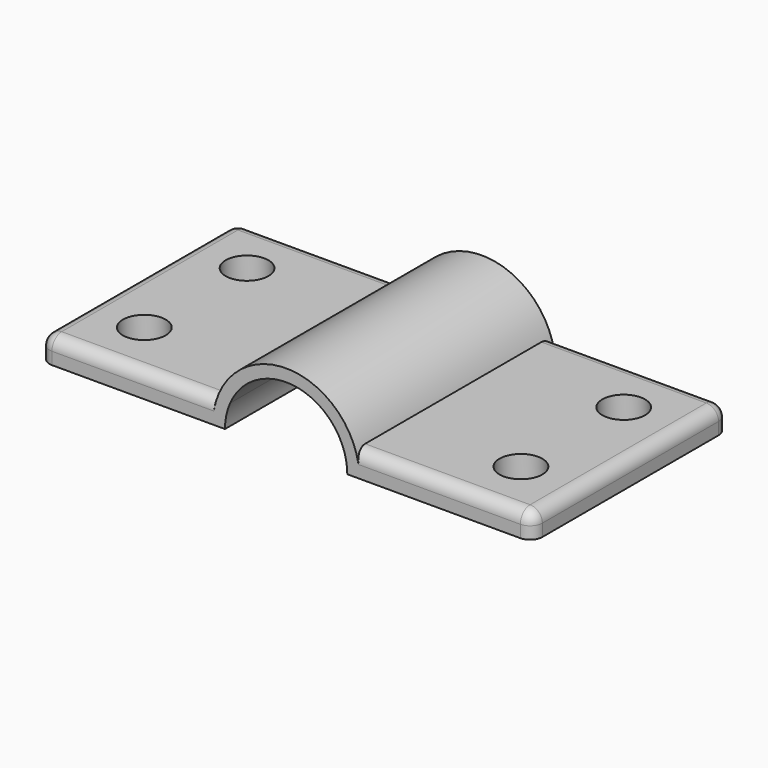
from build123d import *

# Parameters (mm, degrees)
F0_W         = 40.28548
F0_H         = 20
F0_R         = 1.75
F1_DEPTH     = 10
F3_DEPTH     = 25
F4_R         = 1
F5_T1_DEPTH  = 3.5
F5_S5_W      = 1
F5_S5_H      = 1
F5_T6_DEPTH  = 1
F5_S11_W     = 1
F5_S11_H     = 1
F5_T12_DEPTH = 1
F5_S17_W     = 1
F5_S17_H     = 1
F5_T18_DEPTH = 1
F5_S23_W     = 1
F5_S23_H     = 1
F5_T24_DEPTH = 1


# Not quite as in the source:
# - a fillet or chamfer that OpenCascade refuses, or shapes differently, is made with other operations: its cross-section is extruded or revolved along the edge and cut away or added


with BuildPart() as f1:
    # F0 (on Top) → F1 (new body)
    with BuildSketch(Plane.XY):
        Rectangle(F0_W, F0_H)
        with Locations((-15.39274, -5.25)):
            Circle(F0_R, mode=Mode.SUBTRACT)
        with Locations((15.39274, -5.25)):
            Circle(F0_R, mode=Mode.SUBTRACT)
        with Locations((-15.39274, 5.25)):
            Circle(F0_R, mode=Mode.SUBTRACT)
        with Locations((15.39274, 5.25)):
            Circle(F0_R, mode=Mode.SUBTRACT)
    extrude(amount=F1_DEPTH)

    # F2 (on face) → F3 (cut)
    with BuildSketch(Plane.XZ.offset(10)):
        with BuildLine():
            Line((-4.582575695, 2), (4.582575695, 2))
            ThreePointArc((4.582575695, 2), (0, 5), (-4.582575695, 2))
        make_face()
        with BuildLine():
            Line((-5, 0), (5, 0))
            ThreePointArc((5, 0), (4.8945315647, 1.0215482184), (4.582575695, 2))
            Line((4.582575695, 2), (-4.582575695, 2))
            ThreePointArc((-4.582575695, 2), (-4.8945315647, 1.0215482184), (-5, 0))
        make_face()
        with BuildLine():
            ThreePointArc((-5.6568542495, 2), (0, 6), (5.6568542495, 2))
            Line((5.6568542495, 2), (20.14274, 2))
            Line((20.14274, 2), (20.14274, 10))
            Line((20.14274, 10), (-20.14274, 10))
            Line((-20.14274, 10), (-20.14274, 2))
            Line((-20.14274, 2), (-5.6568542495, 2))
        make_face()
    extrude(amount=-F3_DEPTH, mode=Mode.SUBTRACT)

    # F4
    f4_edges = [f1.edges().sort_by_distance(p)[0] for p in [
        (-20.14274, 0, 2),
        (-12.899797, -10, 2),
        (-12.899797, 10, 2),
        (12.899797, 10, 2),
        (20.14274, 0, 2),
        (12.899797, -10, 2),
    ]]
    fillet(f4_edges, radius=F4_R)

    # F5: fillet of radius 1 on 4 edges, made by hand

    # F5_s2 → F5_t1 (cut)
    with BuildSketch(Plane.XY.offset(-2.5)):
        with BuildLine():
            ThreePointArc((20.14274, -9), (19.8498467812, -9.7071067812), (19.14274, -10))
            Line((19.14274, -10), (20.14274, -10))
            Line((20.14274, -10), (20.14274, -9))
        make_face()
        with BuildLine():
            ThreePointArc((19.14274, 10), (19.8498467812, 9.7071067812), (20.14274, 9))
            Line((20.14274, 9), (20.14274, 10))
            Line((20.14274, 10), (19.14274, 10))
        make_face()
        with BuildLine():
            ThreePointArc((-19.14274, 10), (-19.8498467812, 9.7071067812), (-20.14274, 9))
            Line((-20.14274, 9), (-20.14274, 10))
            Line((-20.14274, 10), (-19.14274, 10))
        make_face()
        with BuildLine():
            ThreePointArc((-20.14274, -9), (-19.8498467812, -9.7071067812), (-19.14274, -10))
            Line((-19.14274, -10), (-20.14274, -10))
            Line((-20.14274, -10), (-20.14274, -9))
        make_face()
    extrude(amount=F5_T1_DEPTH, mode=Mode.SUBTRACT)


with BuildPart() as f5_tool4:
    # F5_s5 → F5_t6 (new body)
    with BuildSketch(Plane.YZ.offset(-19.14274)):
        with Locations((-9.5, 1.5)):
            Rectangle(F5_S5_W, F5_S5_H)
    extrude(amount=-F5_T6_DEPTH)

    # F5_s7 → F5_t8 (revolve, cut)
    with BuildSketch(Plane(origin=(-19.14274, -9, 1), x_dir=(0, 0.7071067812, -0.7071067812), z_dir=(0, 0.7071067812, 0.7071067812))):
        with BuildLine():
            ThreePointArc((0, -1), (1, 0), (0, 1))
            Line((0, 1), (0, -1))
        make_face()
    revolve(axis=Axis((-19.14274, -9, 1), (-1, 0, 0)), mode=Mode.SUBTRACT)


with BuildPart() as f1_1:
    add(f1.part)

    # F5_t3: cut F5_tool4
    add(f5_tool4.part, mode=Mode.SUBTRACT)


with BuildPart() as f5_tool10:
    # F5_s11 → F5_t12 (new body)
    with BuildSketch(Plane.XZ.offset(-9)):
        with Locations((-19.64274, 1.5)):
            Rectangle(F5_S11_W, F5_S11_H)
    extrude(amount=-F5_T12_DEPTH)

    # F5_s13 → F5_t14 (revolve, cut)
    with BuildSketch(Plane(origin=(-19.14274, 9, 1), x_dir=(0.7071067812, 0, -0.7071067812), z_dir=(0.7071067812, 0, 0.7071067812))):
        with BuildLine():
            ThreePointArc((0, -1), (1, 0), (0, 1))
            Line((0, 1), (0, -1))
        make_face()
    revolve(axis=Axis((-19.14274, 9, 1), (0, 1, 0)), mode=Mode.SUBTRACT)


with BuildPart() as f1_2:
    add(f1_1.part)

    # F5_t9: cut F5_tool10
    add(f5_tool10.part, mode=Mode.SUBTRACT)


with BuildPart() as f5_tool16:
    # F5_s17 → F5_t18 (new body)
    with BuildSketch(Plane.XZ.offset(-9)):
        with Locations((19.64274, 1.5)):
            Rectangle(F5_S17_W, F5_S17_H)
    extrude(amount=-F5_T18_DEPTH)

    # F5_s19 → F5_t20 (revolve, cut)
    with BuildSketch(Plane(origin=(19.14274, 9, 1), x_dir=(-0.7071067812, 0, -0.7071067812), z_dir=(0.7071067812, 0, -0.7071067812))):
        with BuildLine():
            ThreePointArc((0, -1), (1, 0), (0, 1))
            Line((0, 1), (0, -1))
        make_face()
    revolve(axis=Axis((19.14274, 9, 1), (0, 1, 0)), mode=Mode.SUBTRACT)


with BuildPart() as f1_3:
    add(f1_2.part)

    # F5_t15: cut F5_tool16
    add(f5_tool16.part, mode=Mode.SUBTRACT)


with BuildPart() as f5_tool22:
    # F5_s23 → F5_t24 (new body)
    with BuildSketch(Plane.YZ.offset(19.14274)):
        with Locations((-9.5, 1.5)):
            Rectangle(F5_S23_W, F5_S23_H)
    extrude(amount=F5_T24_DEPTH)

    # F5_s25 → F5_t26 (revolve, cut)
    with BuildSketch(Plane(origin=(19.14274, -9, 1), x_dir=(0, 0.7071067812, -0.7071067812), z_dir=(0, -0.7071067812, -0.7071067812))):
        with BuildLine():
            ThreePointArc((0, -1), (1, 0), (0, 1))
            Line((0, 1), (0, -1))
        make_face()
    revolve(axis=Axis((19.14274, -9, 1), (1, 0, 0)), mode=Mode.SUBTRACT)


with BuildPart() as f1_4:
    add(f1_3.part)

    # F5_t21: cut F5_tool22
    add(f5_tool22.part, mode=Mode.SUBTRACT)


solid = f1_4.part
